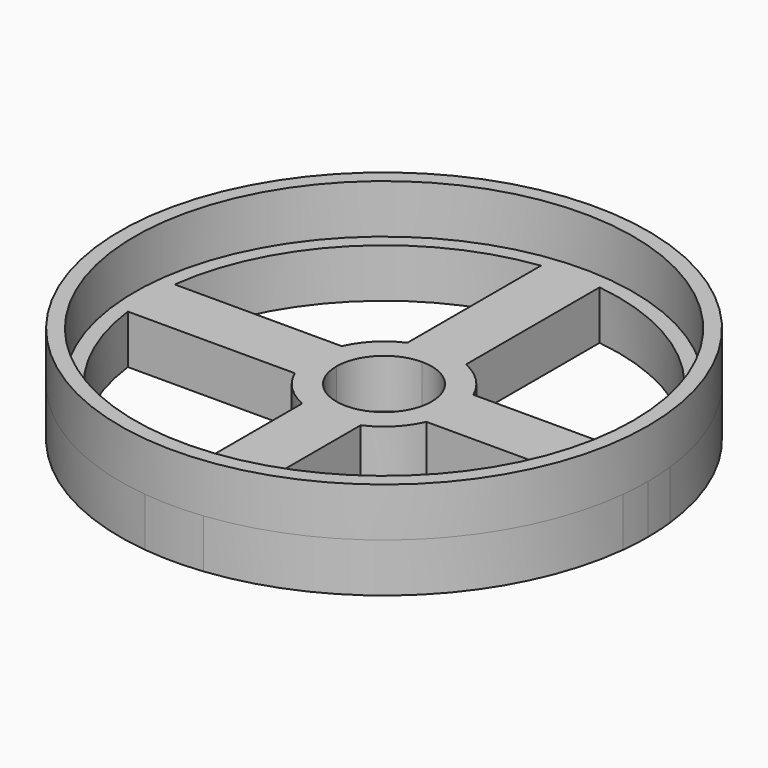
from build123d import *

# Parameters (mm, degrees)
F1_DEPTH = 5
F2_R     = 27
F2_R_2   = 25.5
F3_DEPTH = 5


# Not quite as in the source:
# - a feature names something its author has since deleted; it is built from what else it names


with BuildPart() as f1:
    # F0 (on Top) → F1 (new body)
    with BuildSketch(Plane.XY):
        with BuildLine():
            Line((26.83281573, 3), (23.8117617996, 3))
            ThreePointArc((23.8117617996, 3), (23.9528942217, 1.502949901), (24, 0))
            ThreePointArc((24, 0), (23.9528942217, -1.502949901), (23.8117617996, -3))
            Line((23.8117617996, -3), (26.83281573, -3))
            ThreePointArc((26.83281573, -3), (26.9581715321, -1.5023274094), (27, 0))
            ThreePointArc((27, 0), (26.9581715321, 1.5023274094), (26.83281573, 3))
        make_face()
        with BuildLine():
            ThreePointArc((3, 23.8117617996), (16.9705627485, 16.9705627485), (23.8117617996, 3))
            Line((23.8117617996, 3), (26.83281573, 3))
            ThreePointArc((26.83281573, 3), (19.091883092, 19.091883092), (3, 26.83281573))
            Line((3, 26.83281573), (3, 23.8117617996))
        make_face()
        with BuildLine():
            Line((26.83281573, -3), (23.8117617996, -3))
            ThreePointArc((23.8117617996, -3), (16.9705627485, -16.9705627485), (3, -23.8117617996))
            Line((3, -23.8117617996), (3, -26.83281573))
            ThreePointArc((3, -26.83281573), (19.091883092, -19.091883092), (26.83281573, -3))
        make_face()
        with BuildLine():
            ThreePointArc((-3, 23.8117617996), (0, 24), (3, 23.8117617996))
            Line((3, 23.8117617996), (3, 26.83281573))
            ThreePointArc((3, 26.83281573), (0, 27), (-3, 26.83281573))
            Line((-3, 26.83281573), (-3, 23.8117617996))
        make_face()
        with BuildLine():
            ThreePointArc((-23.8117617996, 3), (-16.9705627485, 16.9705627485), (-3, 23.8117617996))
            Line((-3, 23.8117617996), (-3, 26.83281573))
            ThreePointArc((-3, 26.83281573), (-19.091883092, 19.091883092), (-26.83281573, 3))
            Line((-26.83281573, 3), (-23.8117617996, 3))
        make_face()
        with BuildLine():
            Line((-3, -26.83281573), (-3, -23.8117617996))
            ThreePointArc((-3, -23.8117617996), (-16.9705627485, -16.9705627485), (-23.8117617996, -3))
            Line((-23.8117617996, -3), (-26.83281573, -3))
            ThreePointArc((-26.83281573, -3), (-19.091883092, -19.091883092), (-3, -26.83281573))
        make_face()
        with BuildLine():
            ThreePointArc((3, -23.8117617996), (0, -24), (-3, -23.8117617996))
            Line((-3, -23.8117617996), (-3, -26.83281573))
            ThreePointArc((-3, -26.83281573), (0, -27), (3, -26.83281573))
            Line((3, -26.83281573), (3, -23.8117617996))
        make_face()
        with BuildLine():
            ThreePointArc((-23.8117617996, -3), (-24, 0), (-23.8117617996, 3))
            Line((-23.8117617996, 3), (-26.83281573, 3))
            ThreePointArc((-26.83281573, 3), (-27, 0), (-26.83281573, -3))
            Line((-26.83281573, -3), (-23.8117617996, -3))
        make_face()
        with BuildLine():
            ThreePointArc((-6.7372564891, -3), (-7.2138024511, -1.5335185674), (-7.375, 0))
            ThreePointArc((-7.375, 0), (-7.2138024511, 1.5335185674), (-6.7372564891, 3))
            Line((-6.7372564891, 3), (-23.8117617996, 3))
            ThreePointArc((-23.8117617996, 3), (-24, 0), (-23.8117617996, -3))
            Line((-23.8117617996, -3), (-6.7372564891, -3))
        make_face()
        with BuildLine():
            ThreePointArc((-4.875, 0), (-3.4471455583, 3.4471455583), (0, 4.875))
            Line((0, 4.875), (0, 7.375))
            ThreePointArc((0, 7.375), (-1.5335185674, 7.2138024511), (-3, 6.7372564891))
            ThreePointArc((-3, 6.7372564891), (-5.2149125113, 5.2149125113), (-6.7372564891, 3))
            ThreePointArc((-6.7372564891, 3), (-7.2138024511, 1.5335185674), (-7.375, 0))
            Line((-7.375, 0), (-4.875, 0))
        make_face()
        with BuildLine():
            Line((0, -7.375), (0, -4.875))
            ThreePointArc((0, -4.875), (-3.4471455583, -3.4471455583), (-4.875, 0))
            Line((-4.875, 0), (-7.375, 0))
            ThreePointArc((-7.375, 0), (-7.2138024511, -1.5335185674), (-6.7372564891, -3))
            ThreePointArc((-6.7372564891, -3), (-5.2149125113, -5.2149125113), (-3, -6.7372564891))
            ThreePointArc((-3, -6.7372564891), (-1.5335185674, -7.2138024511), (0, -7.375))
        make_face()
        with BuildLine():
            Line((7.375, 0), (4.875, 0))
            ThreePointArc((4.875, 0), (3.4471455583, -3.4471455583), (0, -4.875))
            Line((0, -4.875), (0, -7.375))
            ThreePointArc((0, -7.375), (1.5335185674, -7.2138024511), (3, -6.7372564891))
            ThreePointArc((3, -6.7372564891), (5.2149125113, -5.2149125113), (6.7372564891, -3))
            ThreePointArc((6.7372564891, -3), (7.2138024511, -1.5335185674), (7.375, 0))
        make_face()
        with BuildLine():
            ThreePointArc((0, 4.875), (3.4471455583, 3.4471455583), (4.875, 0))
            Line((4.875, 0), (7.375, 0))
            ThreePointArc((7.375, 0), (7.2138024511, 1.5335185674), (6.7372564891, 3))
            ThreePointArc((6.7372564891, 3), (5.2149125113, 5.2149125113), (3, 6.7372564891))
            ThreePointArc((3, 6.7372564891), (1.5335185674, 7.2138024511), (0, 7.375))
            Line((0, 7.375), (0, 4.875))
        make_face()
        with BuildLine():
            ThreePointArc((-3, 6.7372564891), (-1.5335185674, 7.2138024511), (0, 7.375))
            ThreePointArc((0, 7.375), (1.5335185674, 7.2138024511), (3, 6.7372564891))
            Line((3, 6.7372564891), (3, 23.8117617996))
            ThreePointArc((3, 23.8117617996), (0, 24), (-3, 23.8117617996))
            Line((-3, 23.8117617996), (-3, 6.7372564891))
        make_face()
        with BuildLine():
            ThreePointArc((6.7372564891, 3), (7.2138024511, 1.5335185674), (7.375, 0))
            ThreePointArc((7.375, 0), (7.2138024511, -1.5335185674), (6.7372564891, -3))
            Line((6.7372564891, -3), (23.8117617996, -3))
            ThreePointArc((23.8117617996, -3), (23.9528942217, -1.502949901), (24, 0))
            ThreePointArc((24, 0), (23.9528942217, 1.502949901), (23.8117617996, 3))
            Line((23.8117617996, 3), (6.7372564891, 3))
        make_face()
        with BuildLine():
            ThreePointArc((3, -6.7372564891), (1.5335185674, -7.2138024511), (0, -7.375))
            ThreePointArc((0, -7.375), (-1.5335185674, -7.2138024511), (-3, -6.7372564891))
            Line((-3, -6.7372564891), (-3, -23.8117617996))
            ThreePointArc((-3, -23.8117617996), (0, -24), (3, -23.8117617996))
            Line((3, -23.8117617996), (3, -6.7372564891))
        make_face()
    extrude(amount=F1_DEPTH)

    # F2 (on face) → F3 (join)
    with BuildSketch(Plane.XY.offset(5)):
        Circle(F2_R)
        Circle(F2_R_2, mode=Mode.SUBTRACT)
    extrude(amount=F3_DEPTH)


solid = f1.part
